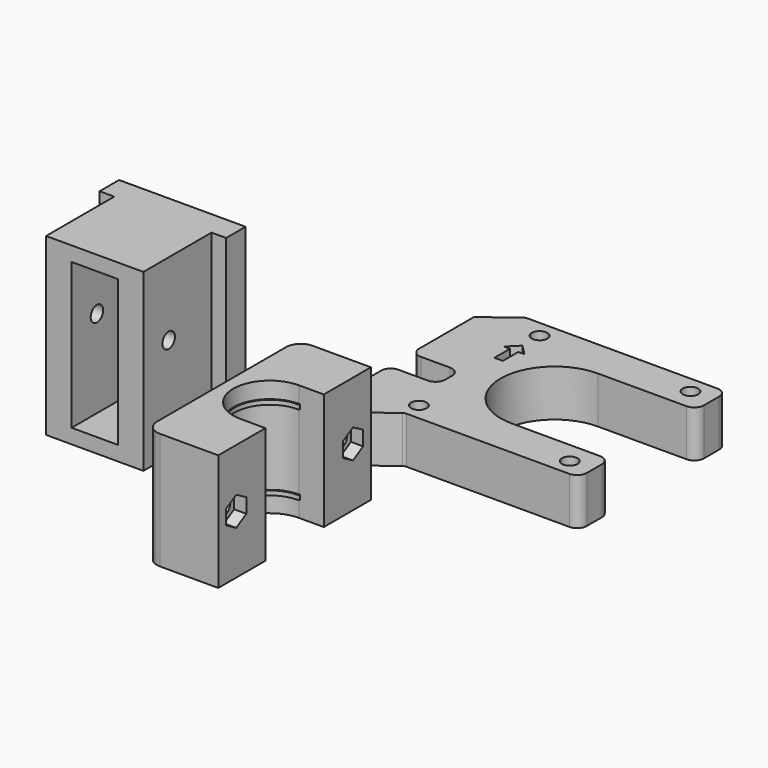
from build123d import *

# Parameters (mm, degrees)
F1_R      = 1.6
F2_DEPTH  = 9.6
F4_DEPTH  = 9.601
F6_DEPTH  = 3.35
F8_DEPTH  = 0.9
F10_DEPTH = 15.5
F12_DEPTH = 0.9
F14_DEPTH = 3.35
F16_DEPTH = 2.5
F17_D     = 3.2
F19_DEPTH = 36
F21_D     = 3.2
F22_W     = 9.5
F22_H     = 30
F23_DEPTH = 17.5
F24_W     = 3.1
F24_H     = 6
F25_DEPTH = 2.5
F26_D     = 3
F26_DEPTH = 6
F26_TIP   = 0.9012909285
F28_DEPTH = 2.5


# Not quite as in the source:
# - ends of sketch curves that miss each other by under 0.0002 mm in the source are joined


with BuildPart() as f2:
    # F1 (on Top) → F2 (new body)
    with BuildSketch(Plane.XY):
        with BuildLine():
            Line((8, 16.124992), (7, 16.124992))
            Line((7, 16.124992), (2.999972, 16.124992))
            Line((2.999972, 16.124992), (2, 16.124992))
            ThreePointArc((2, 16.124992), (0.5857864376, 15.5392055624), (0, 14.124992))
            Line((0, 14.124992), (0, 12.266015))
            Line((0, 12.266015), (3e-06, 4.533969))
            Line((3e-06, 4.533969), (0, 0))
            Line((0, 0), (5.201295, 0))
            ThreePointArc((5.201295, 0), (5.5183912482, 0.0516066378), (5.8027589539, 0.2011000612))
            Line((5.8027589539, 0.2011000612), (11.909819, 4.798899))
            ThreePointArc((11.909819, 4.798899), (12.1916364226, 4.9475355039), (12.5059020779, 4.9999845174))
            ThreePointArc((12.5059020779, 4.9999845174), (12.5085930292, 4.9999953793), (12.511284, 4.999999))
            Line((12.511284, 4.999999), (14.511284, 4.999999))
            Line((14.511284, 4.999999), (45.999966, 4.999999))
            ThreePointArc((45.999966, 4.999999), (47.4141795624, 5.5857854376), (47.999966, 6.999999))
            Line((47.999966, 6.999999), (47.999966, 10.899988))
            ThreePointArc((47.999966, 10.899988), (47.4141795624, 12.3142015624), (45.999966, 12.899988))
            Line((45.999966, 12.899988), (27.783699, 12.899988))
            ThreePointArc((27.783699, 12.899988), (16.683699, 23.999988), (27.783699, 35.099988))
            Line((27.783699, 35.099988), (45.999966, 35.099988))
            ThreePointArc((45.999966, 35.099988), (47.4141795624, 35.6857744376), (47.999966, 37.099988))
            Line((47.999966, 37.099988), (47.999966, 40.999983))
            ThreePointArc((47.999966, 40.999983), (47.4141795624, 42.4141965624), (45.999966, 42.999983))
            Line((45.999966, 42.999983), (8.975639, 42.999983))
            Line((8.975639, 42.999983), (7.1237, 42.999983))
            Line((7.1237, 42.999983), (6.980551, 42.999983))
            Line((6.980551, 42.999983), (6.975639, 42.999983))
            ThreePointArc((6.975639, 42.999983), (6.975435, 42.9999829792), (6.975231, 42.9999829168))
            ThreePointArc((6.975231, 42.9999829168), (6.6583489074, 42.9483115281), (6.3741744079, 42.7988824583))
            Line((6.3741744079, 42.7988824583), (3e-06, 37.999986))
            Line((3e-06, 37.999986), (0, 33.466017))
            Line((0, 33.466017), (3e-06, 25.73397))
            Line((3e-06, 25.73397), (1.9137e-06, 23.8749931687))
            ThreePointArc((1.9137e-06, 23.8749931687), (0.5857879382, 22.4607788508), (2.0000019137, 21.874992))
            Line((2.0000019137, 21.874992), (2.999972, 21.874992))
            Line((2.999972, 21.874992), (7, 21.874992))
            Line((7, 21.874992), (8, 21.874992))
            ThreePointArc((8, 21.874992), (9.4142135624, 21.2892055624), (10, 19.874992))
            Line((10, 19.874992), (10, 18.124992))
            ThreePointArc((10, 18.124992), (9.4142135624, 16.7107784376), (8, 16.124992))
        make_face()
        with Locations((12.283699, 8.499988)):
            Circle(F1_R, mode=Mode.SUBTRACT)
        with Locations((43.283699, 8.499988)):
            Circle(F1_R, mode=Mode.SUBTRACT)
        with Locations((12.283699, 39.499988)):
            Circle(F1_R, mode=Mode.SUBTRACT)
        with Locations((43.283699, 39.499988)):
            Circle(F1_R, mode=Mode.SUBTRACT)
    extrude(amount=F2_DEPTH)

    # F3 (on face) → F4 (cut, through all)
    with BuildSketch(Plane.XY.offset(9.6)):
        Polygon((14.3977755507, 32.9714485153), (12.283699, 35.099988), (10.1551595153, 32.9859114493), (11.4051595153, 32.9859114493), (11.4051595153, 28.9859114493), (13.1477755507, 28.9859114493), (13.1477755507, 32.9714485153), align=None)
    extrude(amount=-F4_DEPTH, mode=Mode.SUBTRACT)


with BuildPart() as f6:
    # F5 (on Top) → F6 (new body)
    with BuildSketch(Plane.XY):
        with BuildLine():
            Line((15.2724227719, -46.7757768929), (15.2724227719, -34.6757708929))
            Line((15.2724227719, -34.6757708929), (10.1734037719, -34.6757708929))
            ThreePointArc((10.1734037719, -34.6757708929), (2.6734037719, -27.1757708929), (10.1734037719, -19.6757708929))
            Line((10.1734037719, -19.6757708929), (15.2724227719, -19.6757708929))
            Line((15.2724227719, -19.6757708929), (15.2724227719, -7.5757648929))
            Line((15.2724227719, -7.5757648929), (3.2636767719, -7.5757648929))
            ThreePointArc((3.2636767719, -7.5757648929), (1.1423564283, -8.4544445493), (0.2636767719, -10.5757648929))
            Line((0.2636767719, -10.5757648929), (0.2636767719, -43.7757768929))
            ThreePointArc((0.2636767719, -43.7757768929), (1.1423564283, -45.8970972365), (3.2636767719, -46.7757768929))
            Line((3.2636767719, -46.7757768929), (15.2724227719, -46.7757768929))
        make_face()
    extrude(amount=F6_DEPTH)

    # F7 (on face) → F8 (join)
    with BuildSketch(Plane.XY.offset(3.35)):
        with BuildLine():
            ThreePointArc((10.1734037719, -34.4257708929), (2.9234037719, -27.1757708929), (10.1734037719, -19.9257708929))
            Line((10.1734037719, -19.9257708929), (10.1734037719, -19.6757708929))
            Line((10.1734037719, -19.6757708929), (10.4234037719, -19.6757708929))
            Line((10.4234037719, -19.6757708929), (15.2724227719, -19.6757708929))
            Line((15.2724227719, -19.6757708929), (15.2724227719, -7.5757648929))
            Line((15.2724227719, -7.5757648929), (3.2636767719, -7.5757648929))
            ThreePointArc((3.2636767719, -7.5757648929), (1.1423564283, -8.4544445493), (0.2636767719, -10.5757648929))
            Line((0.2636767719, -10.5757648929), (0.2636767719, -43.7757768929))
            ThreePointArc((0.2636767719, -43.7757768929), (1.1423564283, -45.8970972365), (3.2636767719, -46.7757768929))
            Line((3.2636767719, -46.7757768929), (15.2724227719, -46.7757768929))
            Line((15.2724227719, -46.7757768929), (15.2724227719, -34.6757708929))
            Line((15.2724227719, -34.6757708929), (10.4234037719, -34.6757708929))
            Line((10.4234037719, -34.6757708929), (10.1734037719, -34.6757708929))
            Line((10.1734037719, -34.6757708929), (10.1734037719, -34.4257708929))
        make_face()
        with BuildLine():
            Line((10.1734037719, -19.6757708929), (10.1734037719, -19.9257708929))
            ThreePointArc((10.1734037719, -19.9257708929), (10.3501804672, -19.8525475882), (10.4234037719, -19.6757708929))
            Line((10.4234037719, -19.6757708929), (10.1734037719, -19.6757708929))
        make_face()
        with BuildLine():
            ThreePointArc((10.4234037719, -34.6757708929), (10.3501804672, -34.4989941976), (10.1734037719, -34.4257708929))
            Line((10.1734037719, -34.4257708929), (10.1734037719, -34.6757708929))
            Line((10.1734037719, -34.6757708929), (10.4234037719, -34.6757708929))
        make_face()
    extrude(amount=F8_DEPTH)

    # F9 (on face) → F10 (join)
    with BuildSketch(Plane.XY.offset(4.25)):
        with BuildLine():
            ThreePointArc((10.1734037719, -34.6757708929), (2.6734037719, -27.1757708929), (10.1734037719, -19.6757708929))
            Line((10.1734037719, -19.6757708929), (15.2724227719, -19.6757708929))
            Line((15.2724227719, -19.6757708929), (15.2724227719, -7.5757648929))
            Line((15.2724227719, -7.5757648929), (3.2636767719, -7.5757648929))
            ThreePointArc((3.2636767719, -7.5757648929), (1.1423564283, -8.4544445493), (0.2636767719, -10.5757648929))
            Line((0.2636767719, -10.5757648929), (0.2636767719, -43.7757768929))
            ThreePointArc((0.2636767719, -43.7757768929), (1.1423564283, -45.8970972365), (3.2636767719, -46.7757768929))
            Line((3.2636767719, -46.7757768929), (15.2724227719, -46.7757768929))
            Line((15.2724227719, -46.7757768929), (15.2724227719, -34.6757708929))
            Line((15.2724227719, -34.6757708929), (10.1734037719, -34.6757708929))
        make_face()
    extrude(amount=F10_DEPTH)

    # F11 (on face) → F12 (join)
    with BuildSketch(Plane.XY.offset(19.75)):
        with BuildLine():
            ThreePointArc((10.1734037719, -34.4257708929), (2.9234037719, -27.1757708929), (10.1734037719, -19.9257708929))
            ThreePointArc((10.1734037719, -19.9257708929), (10.3501804672, -19.8525475882), (10.4234037719, -19.6757708929))
            Line((10.4234037719, -19.6757708929), (15.2724227719, -19.6757708929))
            Line((15.2724227719, -19.6757708929), (15.2724227719, -7.5757648929))
            Line((15.2724227719, -7.5757648929), (3.2636767719, -7.5757648929))
            ThreePointArc((3.2636767719, -7.5757648929), (1.1423564283, -8.4544445493), (0.2636767719, -10.5757648929))
            Line((0.2636767719, -10.5757648929), (0.2636767719, -43.7757768929))
            ThreePointArc((0.2636767719, -43.7757768929), (1.1423564283, -45.8970972365), (3.2636767719, -46.7757768929))
            Line((3.2636767719, -46.7757768929), (15.2724227719, -46.7757768929))
            Line((15.2724227719, -46.7757768929), (15.2724227719, -34.6757708929))
            Line((15.2724227719, -34.6757708929), (10.4234037719, -34.6757708929))
            ThreePointArc((10.4234037719, -34.6757708929), (10.3501804672, -34.4989941976), (10.1734037719, -34.4257708929))
        make_face()
    extrude(amount=F12_DEPTH)

    # F13 (on face) → F14 (join)
    with BuildSketch(Plane.XY.offset(20.65)):
        with BuildLine():
            ThreePointArc((10.1734037719, -34.6757708929), (2.6734037719, -27.1757708929), (10.1734037719, -19.6757708929))
            Line((10.1734037719, -19.6757708929), (15.2724227719, -19.6757708929))
            Line((15.2724227719, -19.6757708929), (15.2724227719, -7.5757648929))
            Line((15.2724227719, -7.5757648929), (3.2636767719, -7.5757648929))
            ThreePointArc((3.2636767719, -7.5757648929), (1.1423564283, -8.4544445493), (0.2636767719, -10.5757648929))
            Line((0.2636767719, -10.5757648929), (0.2636767719, -43.7757768929))
            ThreePointArc((0.2636767719, -43.7757768929), (1.1423564283, -45.8970972365), (3.2636767719, -46.7757768929))
            Line((3.2636767719, -46.7757768929), (15.2724227719, -46.7757768929))
            Line((15.2724227719, -46.7757768929), (15.2724227719, -34.6757708929))
            Line((15.2724227719, -34.6757708929), (10.1734037719, -34.6757708929))
        make_face()
    extrude(amount=F14_DEPTH)

    # F15 (on face) → F16 (cut)
    with BuildSketch(Plane.YZ.offset(15.2724227719)):
        Polygon((-39.5776946815, 13.5), (-42.1757708929, 15), (-44.7738471043, 13.5), (-44.7738471043, 10.5), (-42.1757708929, 9), (-39.5776946815, 10.5), align=None)
        Polygon((-9.5776946815, 13.5), (-12.1757708929, 15), (-14.7738471043, 13.5), (-14.7738471043, 10.5), (-12.1757708929, 9), (-9.5776946815, 10.5), align=None)
    extrude(amount=-F16_DEPTH, mode=Mode.SUBTRACT)

    # F17 (through all)
    with Locations(Plane.YZ.offset(15.2724227719)):
        with Locations((-42.1757708929, 12), (-12.1757708929, 12)):
            Hole(F17_D / 2)


with BuildPart() as f19:
    # F18 (on Top) → F19 (new body)
    with BuildSketch(Plane.XY):
        Polygon((-16.5402969122, -5), (-16.5402969122, 0), (-42.5402969122, 0), (-42.5402969122, -5), (-39.5402969122, -5), (-39.5402969122, -22.5), (-19.5402969122, -22.5), (-19.5402969122, -5), align=None)
    extrude(amount=F19_DEPTH)

    # F21 (through all)
    with Locations(Plane(origin=(-39.5402969122, 0, 0), x_dir=(0, -1, 0), z_dir=(-1, 0, 0))):
        with Locations((16, 21)):
            Hole(F21_D / 2)

    # F22 (on face) → F23 (cut)
    with BuildSketch(Plane.XZ.offset(22.5)):
        with Locations((-29.5402969122, 18)):
            Rectangle(F22_W, F22_H)
    extrude(amount=-F23_DEPTH, mode=Mode.SUBTRACT)

    # F24 (on face) → F25 (join)
    with BuildSketch(Plane(origin=(0, 0, 0), x_dir=(-1, 0, 0), z_dir=(0, 1, 0))):
        with Locations((23.2402969122, 27.9)):
            Rectangle(F24_W, F24_H)
        with Locations((35.8402969122, 27.9)):
            Rectangle(F24_W, F24_H)
        with Locations((23.2402969122, 6.7)):
            Rectangle(F24_W, F24_H)
        with Locations((35.8402969122, 6.7)):
            Rectangle(F24_W, F24_H)
    extrude(amount=F25_DEPTH)

    # F26
    with Locations(Plane(origin=(0, 0, 0), x_dir=(-1, 0, 0), z_dir=(0, 1, 0))):
        with Locations((23.2402969122, 17.3), (35.8402969122, 17.3)):
            Hole(F26_D / 2, depth=F26_DEPTH)
            with Locations((0, 0, -(F26_DEPTH + F26_TIP / 2))):  # 118° drill point
                Cone(0, F26_D / 2, F26_TIP, mode=Mode.SUBTRACT)

    # F27 (on face) → F28 (cut)
    with BuildSketch(Plane(origin=(0, 0, 0), x_dir=(-1, 0, 0), z_dir=(0, 1, 0))):
        Polygon((24.6836725852, 19.8), (21.7969212392, 19.8), (20.3535455662, 17.3), (21.7969212392, 14.8), (24.6836725852, 14.8), (26.1270482581, 17.3), align=None)
        Polygon((37.2836725852, 19.8), (34.3969212392, 19.8), (32.9535455662, 17.3), (34.3969212392, 14.8), (37.2836725852, 14.8), (38.7270482581, 17.3), align=None)
    extrude(amount=-F28_DEPTH, mode=Mode.SUBTRACT)


solid = Compound([f2.part, f6.part, f19.part])
